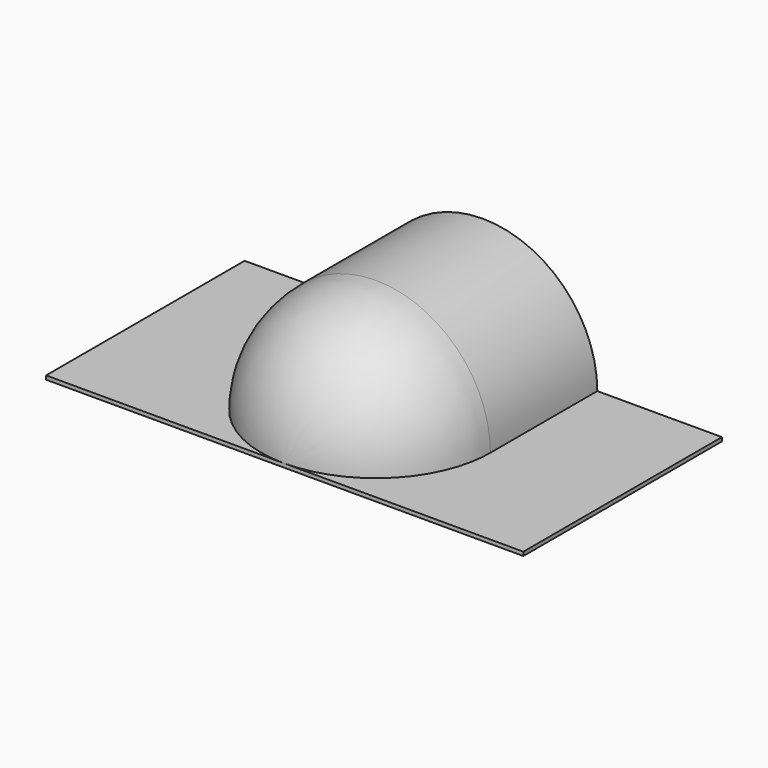
from build123d import *

# Parameters (mm, degrees)
F0_W     = 250
F0_H     = 130
F2_DEPTH = 2
F3_DEPTH = 130
F4_R     = 59.99999
F6_DEPTH = 47


# Not quite as in the source:
# - a fillet or chamfer is up to 0.001 mm smaller than in the source, because OpenCascade refuses the exact size


with BuildPart() as f2:
    # F0 (on Top) → F2 (new body)
    with BuildSketch(Plane.XY):
        with Locations((-125, -65)):
            Rectangle(F0_W, F0_H)
    extrude(amount=-F2_DEPTH)

    # F1 (on Front) → F3 (join)
    with BuildSketch(Plane.XZ):
        with BuildLine():
            Line((-67.4997093476, 0), (-65.2703463938, 0))
            ThreePointArc((-65.2703463938, 0), (-125.2703463938, 60), (-185.2703463938, 0))
            Line((-185.2703463938, 0), (-183.04098344, 0))
            ThreePointArc((-183.04098344, 0), (-125.2703463938, 57.7706370462), (-67.4997093476, 0))
        make_face()
        with BuildLine():
            Line((-183.04098344, 0), (-67.4997093476, 0))
            ThreePointArc((-67.4997093476, 0), (-125.2703463938, 57.7706370462), (-183.04098344, 0))
        make_face()
    extrude(amount=F3_DEPTH)

    # F4 (radius 60 in the source; OpenCascade refuses exactly that, so slightly less here)
    f4_edges = [f2.edges().sort_by_distance(p)[0] for p in [
        (-125.270346, -130, 60),
    ]]
    fillet(f4_edges, radius=F4_R)

    # F5 (on Front) → F6 (cut)
    with BuildSketch(Plane.XZ):
        with BuildLine():
            Line((-183.5164714, 0), (-66.640497432, 0))
            ThreePointArc((-66.640497432, 0), (-125.078484416, 58.437986984), (-183.5164714, 0))
        make_face()
    extrude(amount=F6_DEPTH, mode=Mode.SUBTRACT)


solid = f2.part
